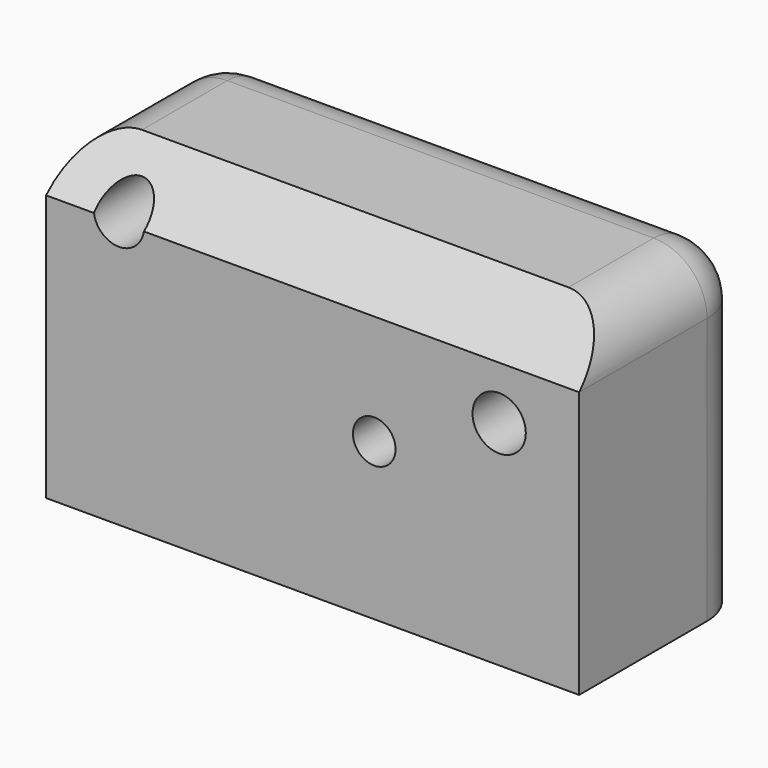
from build123d import *

# Parameters (mm, degrees)
F0_W        = 127
F0_H        = 76.2
F0_R        = 6.0082051914
F0_R_2      = 6.35
F1_DEPTH    = 50.8
F2_R        = 5.0727698676
F3_DEPTH    = 72.136
F4_T1_DEPTH = 192.3207478943
F5_T1_DEPTH = 190.5
F6_T1_DEPTH = 57.15
F6_T3_DEPTH = 95.25
F6_T6_ANGLE = 90.000000001
F6_T8_ANGLE = 90.000000001


# Not quite as in the source:
# - a fillet or chamfer that OpenCascade refuses, or shapes differently, is made with other operations: its cross-section is extruded or revolved along the edge and cut away or added


with BuildPart() as f1:
    # F0 (on Front) → F1 (new body)
    with BuildSketch(Plane.XZ):
        with Locations((-14.6853402257, 47.3040914883)):
            Rectangle(F0_W, F0_H)
        with Locations((-60.8313269913, 73.5488906503)):
            Circle(F0_R, mode=Mode.SUBTRACT)
        with Locations((29.7646597743, 60.0040914883)):
            Circle(F0_R_2, mode=Mode.SUBTRACT)
    extrude(amount=F1_DEPTH)

    # F2 (on face) → F3 (cut)
    with BuildSketch(Plane.XZ.offset(50.8)):
        with Locations((0, 46.5039759874)):
            Circle(F2_R)
    extrude(amount=-F3_DEPTH, mode=Mode.SUBTRACT)

    # F4: chamfer of 12.7 on 1 edges, made by hand

    # F4_s2 → F4_t1 (cut)
    with BuildSketch(Plane.YZ.offset(-110.8457141729)):
        Polygon((-38.1, 85.4040914883), (-50.8, 72.7040914883), (-50.8, 85.4040914883), align=None)
    extrude(amount=F4_T1_DEPTH, mode=Mode.SUBTRACT)

    # F5: fillet of radius 12.7 on 1 edges, made by hand

    # F5_s2 → F5_t1 (cut)
    with BuildSketch(Plane.YZ.offset(-109.9353402257)):
        with BuildLine():
            ThreePointArc((0, 72.7040914883), (-3.7197438789, 81.6843476094), (-12.7, 85.4040914883))
            Line((-12.7, 85.4040914883), (0, 85.4040914883))
            Line((0, 85.4040914883), (0, 72.7040914883))
        make_face()
    extrude(amount=F5_T1_DEPTH, mode=Mode.SUBTRACT)

    # F6: fillet of radius 12.7 on 2 edges, made by hand

    # F6_s2 → F6_t1 (cut)
    with BuildSketch(Plane.XZ.offset(12.7)):
        with BuildLine():
            ThreePointArc((-65.4853402257, 85.4040914883), (-74.4655963468, 81.6843476094), (-78.1853402257, 72.7040914883))
            Line((-78.1853402257, 72.7040914883), (-78.1853402257, 85.4040914883))
            Line((-78.1853402257, 85.4040914883), (-65.4853402257, 85.4040914883))
        make_face()
        with BuildLine():
            ThreePointArc((48.8146597743, 72.7040914883), (45.0949158954, 81.6843476094), (36.1146597743, 85.4040914883))
            Line((36.1146597743, 85.4040914883), (48.8146597743, 85.4040914883))
            Line((48.8146597743, 85.4040914883), (48.8146597743, 72.7040914883))
        make_face()
    extrude(amount=F6_T1_DEPTH, mode=Mode.SUBTRACT)

    # F6_s4 → F6_t3 (cut)
    with BuildSketch(Plane.XY.offset(-22.5459085117)):
        with BuildLine():
            ThreePointArc((48.8146597743, -12.7), (45.0949158954, -3.7197438789), (36.1146597743, 0))
            Line((36.1146597743, 0), (48.8146597743, 0))
            Line((48.8146597743, 0), (48.8146597743, -12.7))
        make_face()
        with BuildLine():
            ThreePointArc((-65.4853402257, 0), (-74.4655963468, -3.7197438789), (-78.1853402257, -12.7))
            Line((-78.1853402257, -12.7), (-78.1853402257, 0))
            Line((-78.1853402257, 0), (-65.4853402257, 0))
        make_face()
    extrude(amount=F6_T3_DEPTH, mode=Mode.SUBTRACT)

    # F6_s5 → F6_t6 (revolve, cut)
    with BuildSketch(Plane.XZ.offset(12.6999999999)):
        with BuildLine():
            ThreePointArc((48.8146597743, 72.7040914883), (45.0949158954, 81.6843476094), (36.1146597743, 85.4040914883))
            Line((36.1146597743, 85.4040914883), (48.8146597743, 85.4040914883))
            Line((48.8146597743, 85.4040914883), (48.8146597743, 72.7040914883))
        make_face()
    revolve(axis=Axis((48.8146597743, -12.6999999999, 72.7040914884), (-1, 0, 0)), revolution_arc=F6_T6_ANGLE, mode=Mode.SUBTRACT)

    # F6_s7 → F6_t8 (revolve, cut)
    with BuildSketch(Plane.XZ.offset(12.6999999999)):
        with BuildLine():
            ThreePointArc((-65.4853402257, 85.4040914883), (-74.4655963468, 81.6843476094), (-78.1853402257, 72.7040914883))
            Line((-78.1853402257, 72.7040914883), (-78.1853402257, 85.4040914883))
            Line((-78.1853402257, 85.4040914883), (-65.4853402257, 85.4040914883))
        make_face()
    revolve(axis=Axis((-78.1853402257, -12.6999999999, 72.7040914884), (-1, 0, 0)), revolution_arc=F6_T8_ANGLE, mode=Mode.SUBTRACT)


solid = f1.part
